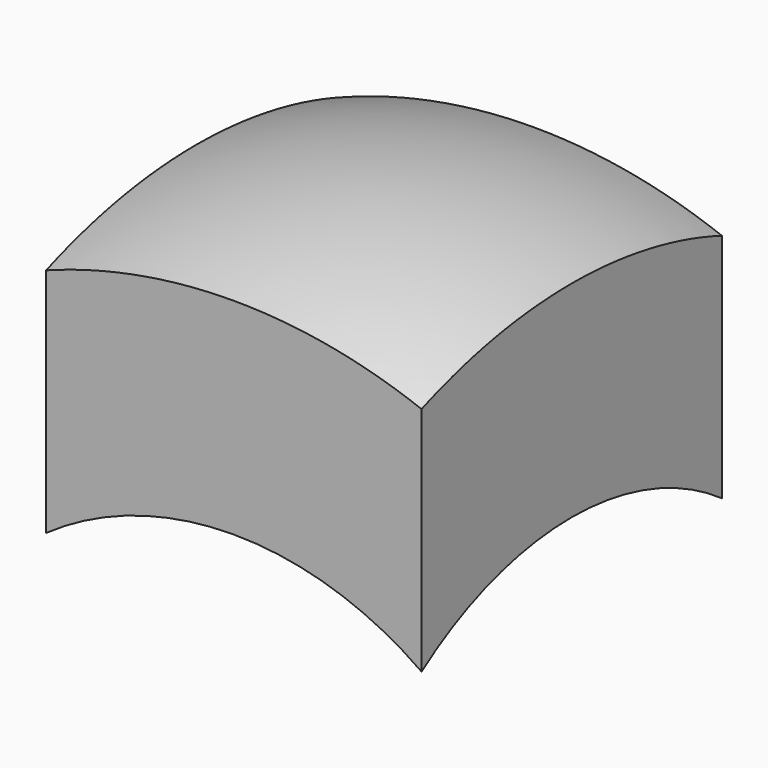
from build123d import *

# Parameters (mm, degrees)
F4_DEPTH = 127
F3_W     = 50.8
F3_H     = 50.8
F5_DEPTH = 127


with BuildPart() as f1:
    # F0 (on Front) → F1 (revolve)
    with BuildSketch(Plane.XZ):
        with BuildLine():
            Line((0, 0), (0, -76.2))
            ThreePointArc((0, -76.2), (76.2, 0), (0, 76.2))
            Line((0, 76.2), (0, 0))
        make_face()
    revolve(axis=Axis((0, 0, 0), (0, 0, -1)))

    # F2 (on Front) → F4 (cut, symmetric)
    with BuildSketch(Plane.XZ):
        with BuildLine():
            Line((-25.4, 25.4), (-25.4, 71.8420489686))
            ThreePointArc((-25.4, 71.8420489686), (-53.8815367264, 53.8815367264), (-71.8420489686, 25.4))
            Line((-71.8420489686, 25.4), (-25.4, 25.4))
        make_face()
        with BuildLine():
            Line((-25.4, -25.4), (-25.4, 25.4))
            Line((-25.4, 25.4), (-71.8420489686, 25.4))
            ThreePointArc((-71.8420489686, 25.4), (-76.2, 0), (-71.8420489686, -25.4))
            Line((-71.8420489686, -25.4), (-25.4, -25.4))
        make_face()
        with BuildLine():
            ThreePointArc((-71.8420489686, -25.4), (-53.8815367264, -53.8815367264), (-25.4, -71.8420489686))
            Line((-25.4, -71.8420489686), (-25.4, -25.4))
            Line((-25.4, -25.4), (-71.8420489686, -25.4))
        make_face()
        with BuildLine():
            ThreePointArc((-25.4, -71.8420489686), (0, -76.2), (25.4, -71.8420489686))
            Line((25.4, -71.8420489686), (25.4, -25.4))
            Line((25.4, -25.4), (-25.4, -25.4))
            Line((-25.4, -25.4), (-25.4, -71.8420489686))
        make_face()
        with BuildLine():
            ThreePointArc((25.4, -71.8420489686), (53.8815367264, -53.8815367264), (71.8420489686, -25.4))
            Line((71.8420489686, -25.4), (25.4, -25.4))
            Line((25.4, -25.4), (25.4, -71.8420489686))
        make_face()
        with BuildLine():
            ThreePointArc((71.8420489686, -25.4), (75.1026102456, -12.8855707789), (76.2, 0))
            ThreePointArc((76.2, 0), (75.1026102456, 12.8855707789), (71.8420489686, 25.4))
            Line((71.8420489686, 25.4), (25.4, 25.4))
            Line((25.4, 25.4), (25.4, -25.4))
            Line((25.4, -25.4), (71.8420489686, -25.4))
        make_face()
        with BuildLine():
            Line((25.4, 25.4), (71.8420489686, 25.4))
            ThreePointArc((71.8420489686, 25.4), (53.8815367264, 53.8815367264), (25.4, 71.8420489686))
            Line((25.4, 71.8420489686), (25.4, 25.4))
        make_face()
    extrude(amount=F4_DEPTH, both=True, mode=Mode.SUBTRACT)

    # F3 (on Right) → F5 (cut, symmetric)
    with BuildSketch(Plane.YZ):
        with BuildLine():
            ThreePointArc((71.8420489686, -25.4), (75.1026102456, -12.8855707789), (76.2, 0))
            ThreePointArc((76.2, 0), (75.1026102456, 12.8855707789), (71.8420489686, 25.4))
            Line((71.8420489686, 25.4), (25.4, 25.4))
            Line((25.4, 25.4), (25.4, -25.4))
            Line((25.4, -25.4), (71.8420489686, -25.4))
        make_face()
        with BuildLine():
            Line((25.4, 25.4), (71.8420489686, 25.4))
            ThreePointArc((71.8420489686, 25.4), (53.8815367264, 53.8815367264), (25.4, 71.8420489686))
            Line((25.4, 71.8420489686), (25.4, 25.4))
        make_face()
        Rectangle(F3_W, F3_H)
        with BuildLine():
            ThreePointArc((-25.4, -71.8420489686), (0, -76.2), (25.4, -71.8420489686))
            Line((25.4, -71.8420489686), (25.4, -25.4))
            Line((25.4, -25.4), (-25.4, -25.4))
            Line((-25.4, -25.4), (-25.4, -71.8420489686))
        make_face()
        with BuildLine():
            Line((-25.4, 25.4), (-25.4, 71.8420489686))
            ThreePointArc((-25.4, 71.8420489686), (-53.8815367264, 53.8815367264), (-71.8420489686, 25.4))
            Line((-71.8420489686, 25.4), (-25.4, 25.4))
        make_face()
        with BuildLine():
            Line((-25.4, -25.4), (-25.4, 25.4))
            Line((-25.4, 25.4), (-71.8420489686, 25.4))
            ThreePointArc((-71.8420489686, 25.4), (-76.2, 0), (-71.8420489686, -25.4))
            Line((-71.8420489686, -25.4), (-25.4, -25.4))
        make_face()
    extrude(amount=F5_DEPTH, both=True, mode=Mode.SUBTRACT)

    # F6 (on Front) → F7 (revolve, cut)
    with BuildSketch(Plane.XZ):
        with BuildLine():
            Line((0, 0), (50.8, 0))
            ThreePointArc((50.8, 0), (0, 50.8), (-50.8, 0))
            Line((-50.8, 0), (0, 0))
        make_face()
    revolve(axis=Axis((25.4, 0, 0), (1, 0, 0)), mode=Mode.SUBTRACT)


solid = f1.part
